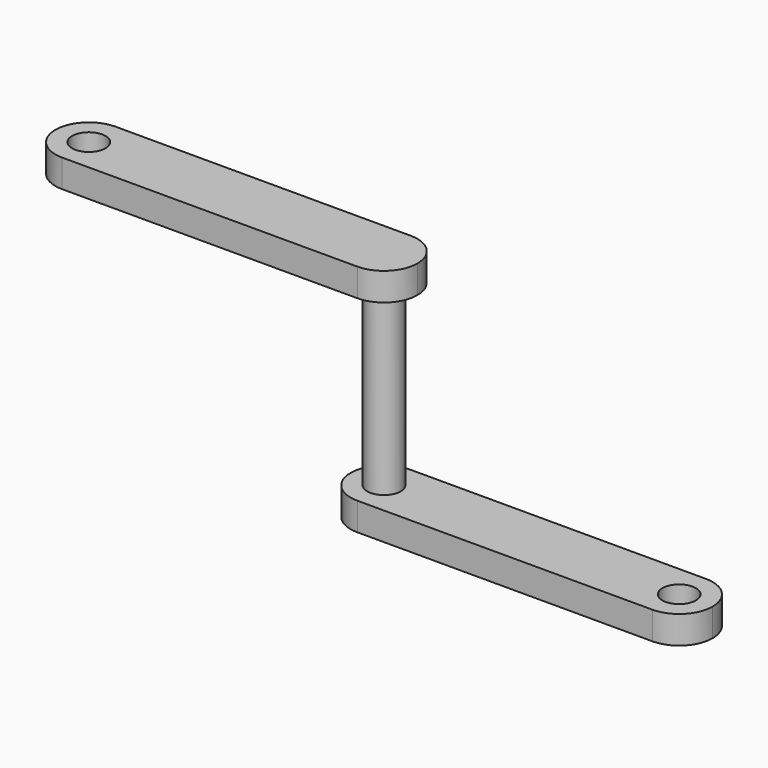
from build123d import *

# Parameters (mm, degrees)
F0_W     = 206.375
F0_H     = 15.875
F1_DEPTH = 38.1
F2_R     = 19.04999
F3_R     = 19.04999
F4_R     = 9.525
F5_DEPTH = 101.6
F6_R     = 9.525
F7_DEPTH = 25.4
F8_R     = 9.525
F9_DEPTH = 25.4


# Not quite as in the source:
# - a fillet or chamfer is up to 0.001 mm smaller than in the source, because OpenCascade refuses the exact size


with BuildPart() as f1:
    # F0 (on Front) → F1 (new body)
    with BuildSketch(Plane.XZ):
        with Locations((103.1875, -7.9375)):
            Rectangle(F0_W, F0_H)
    extrude(amount=F1_DEPTH)

    # F3 (radius 19.05 in the source; OpenCascade refuses exactly that, so slightly less here)
    f3_edges = [f1.edges().sort_by_distance(p)[0] for p in [
        (0, -38.1, -7.9375),
        (206.375, -38.1, -7.9375),
        (206.375, 0, -7.9375),
        (0, 0, -7.9375),
    ]]
    fillet(f3_edges, radius=F3_R)



with BuildPart() as f1b:
    # F0 (on Front) → F1, piece 2 (new body)
    with BuildSketch(Plane.XZ):
        with Locations((-65.0875, 109.5375)):
            Rectangle(F0_W, F0_H)
    extrude(amount=F1_DEPTH)

    # F2 (radius 19.05 in the source; OpenCascade refuses exactly that, so slightly less here)
    f2_edges = [f1b.edges().sort_by_distance(p)[0] for p in [
        (-168.275, -38.1, 109.5375),
        (-168.275, 0, 109.5375),
        (38.1, -38.1, 109.5375),
        (38.1, 0, 109.5375),
    ]]
    fillet(f2_edges, radius=F2_R)


with BuildPart() as f1_1:
    add(f1.part)

    add(f1b.part)  # F5 merges F1b
    # F4 (on face) → F5 (join)
    with BuildSketch(Plane(origin=(0, 0, 101.6), x_dir=(1, 0, 0), z_dir=(0, 0, -1))):
        with Locations((19.05, 19.05)):
            Circle(F4_R)
    extrude(amount=F5_DEPTH)

    # F6 (on face) → F7 (cut)
    with BuildSketch(Plane(origin=(0, 0, 101.6), x_dir=(1, 0, 0), z_dir=(0, 0, -1))):
        with Locations((-149.225, 19.05)):
            Circle(F6_R)
    extrude(amount=-F7_DEPTH, mode=Mode.SUBTRACT)

    # F8 (on face) → F9 (cut)
    with BuildSketch(Plane(origin=(0, 0, -15.875), x_dir=(1, 0, 0), z_dir=(0, 0, -1))):
        with Locations((187.325, 19.05)):
            Circle(F8_R)
    extrude(amount=-F9_DEPTH, mode=Mode.SUBTRACT)


solid = f1_1.part
